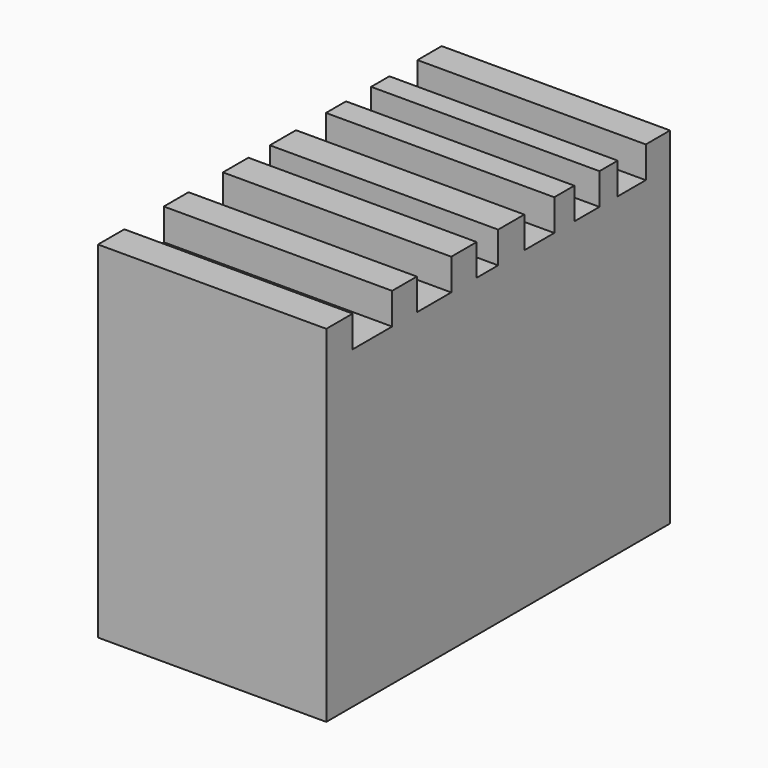
from build123d import *

# Parameters (mm, degrees)
F0_W     = 5.5
F0_H     = 16.3
F0_W_2   = 2.3349355608
F0_H_2   = 2.2036070004
F1_DEPTH = 15
F2_DEPTH = 12
F3_W     = 10.8860824257
F3_H     = 1.5700478107
F3_H_2   = 1.4735469595
F3_H_3   = 1.5152581036
F3_H_4   = 1.5589032643
F3_H_5   = 1.1953348294
F3_H_6   = 1.0883370414
F3_H_7   = 1.4443685184
F4_DEPTH = 1.5


with BuildPart() as f1:
    # F0 (on Top) → F1 (new body)
    with BuildSketch(Plane.XY):
        with Locations((-19.2246585935, -7.1874150395)):
            Rectangle(F0_W, F0_H)
        Polygon((-14.1397230327, 0.9625849605), (-16.4746585935, 0.9625849605), (-16.4746585935, -15.3374150395), (-16.4746585935, -15.3418527916), (-14.1397230327, -15.3418527916), align=None)
        Polygon((-16.4746585935, -15.3374150395), (-21.9746585935, -15.3374150395), (-21.9746585935, -17.545459792), (-16.4746585935, -17.545459792), (-16.4746585935, -15.3418527916), align=None)
        Polygon((-11.0885761678, 0.9625849605), (-14.1397230327, 0.9625849605), (-14.1397230327, -15.3418527916), (-14.1397230327, -17.545459792), (-11.0885761678, -17.545459792), align=None)
        Polygon((-16.4746585935, -17.545459792), (-21.9746585935, -17.545459792), (-21.9746585935, -19.5230543613), (-11.0885761678, -19.5230543613), (-11.0885761678, -17.545459792), (-14.1397230327, -17.545459792), align=None)
        with Locations((-15.3071908131, -16.4436562918)):
            Rectangle(F0_W_2, F0_H_2)
    extrude(amount=F1_DEPTH)

    # F0 (on Top) → F2 (cut)
    with BuildSketch(Plane.XY):
        Polygon((-14.1397230327, 0.9625849605), (-16.4746585935, 0.9625849605), (-16.4746585935, -15.3374150395), (-16.4746585935, -15.3418527916), (-14.1397230327, -15.3418527916), align=None)
        with Locations((-19.2246585935, -7.1874150395)):
            Rectangle(F0_W, F0_H)
        Polygon((-16.4746585935, -15.3374150395), (-21.9746585935, -15.3374150395), (-21.9746585935, -17.545459792), (-16.4746585935, -17.545459792), (-16.4746585935, -15.3418527916), align=None)
        with Locations((-15.3071908131, -16.4436562918)):
            Rectangle(F0_W_2, F0_H_2)
    extrude(amount=F2_DEPTH, mode=Mode.SUBTRACT)

    # F3 (on face) → F4 (join)
    with BuildSketch(Plane.XY.offset(15)):
        with Locations((-16.5316173807, -18.738030456)):
            Rectangle(F3_W, F3_H)
        with Locations((-16.5316173807, -14.8630174808)):
            Rectangle(F3_W, F3_H_2)
        with Locations((-16.5316173807, -11.318010278)):
            Rectangle(F3_W, F3_H_3)
        with Locations((-16.5316173807, -8.5007830683)):
            Rectangle(F3_W, F3_H_4)
        with Locations((-16.5316173807, -5.3385491483)):
            Rectangle(F3_W, F3_H_5)
        with Locations((-16.5316173807, -2.6988773607)):
            Rectangle(F3_W, F3_H_6)
        with Locations((-16.5316173807, 0.2404007013)):
            Rectangle(F3_W, F3_H_7)
    extrude(amount=F4_DEPTH)


solid = f1.part
